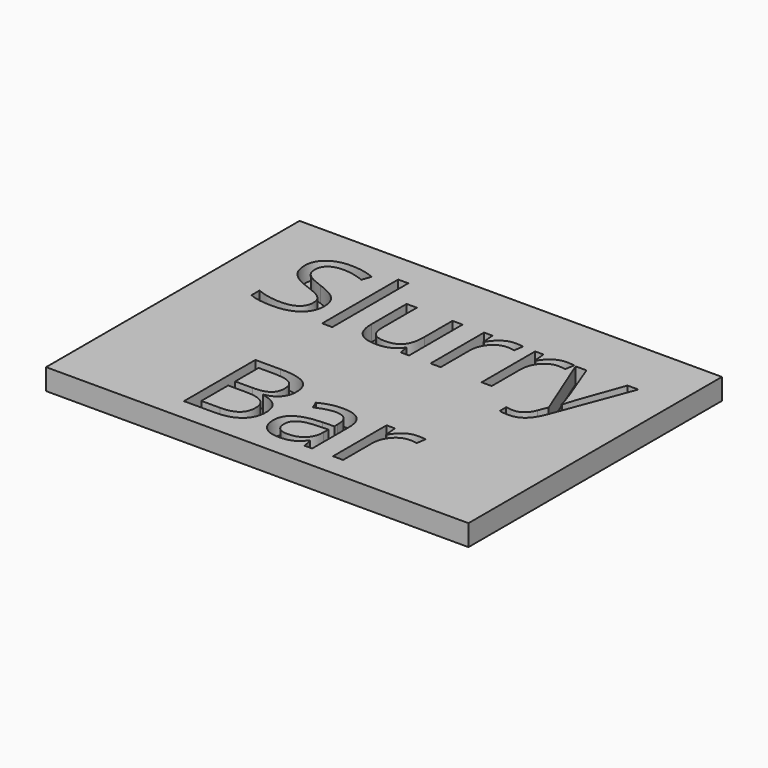
from build123d import *

# Parameters (mm, degrees)
F0_W         = 80
F0_H         = 60
F1_DEPTH     = 4
F2_TEXT_SIZE = 23.6863063441
F3_DEPTH     = 3


# Not quite as in the source:
# - Text() gives the source's letters only with a copy of the font that has no kerning and outlines rounded to 1/6400 em; it was checked with that copy


with BuildPart() as f1:
    # F0 (on Top) → F1 (new body)
    with BuildSketch(Plane.XY):
        with Locations((-1.2539830059, -8.3545163072)):
            Rectangle(F0_W, F0_H)
    extrude(amount=-F1_DEPTH)

    # F2 (on Top) → F3 (cut)
    with BuildSketch(Plane.XY):
        with Locations((-33.1608288818, -1.91181025)):
            Text('Slurry', F2_TEXT_SIZE, font='Open Sans', text_align=(TextAlign.LEFT, TextAlign.BOTTOM))
        with Locations((-20.8513515536, -34.125186878)):
            Text('Bar', F2_TEXT_SIZE, font='Open Sans', text_align=(TextAlign.LEFT, TextAlign.BOTTOM))
    extrude(amount=-F3_DEPTH, mode=Mode.SUBTRACT)


solid = f1.part
